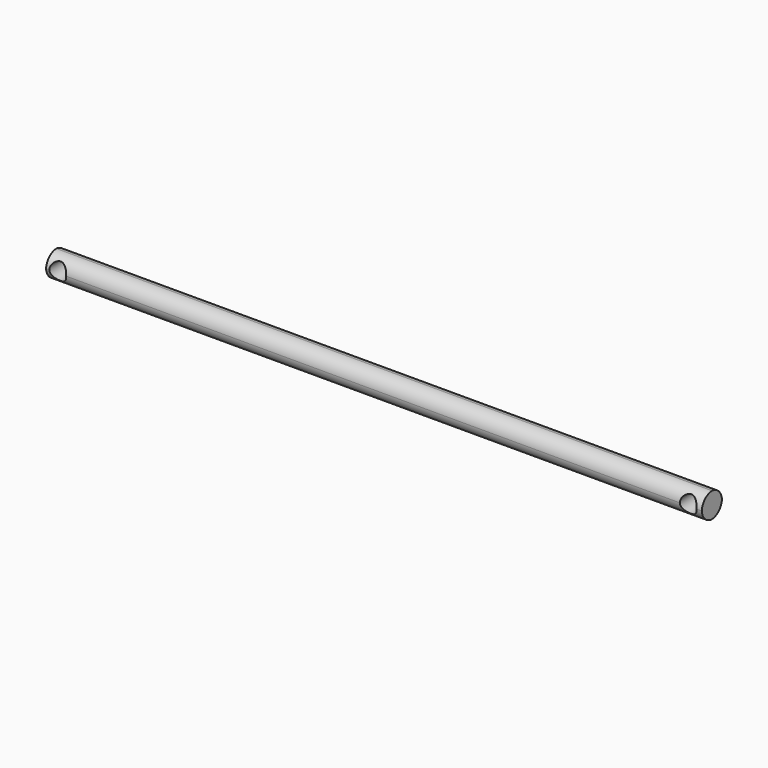
from build123d import *

# Parameters (mm, degrees)
F0_W        = 390
F0_H        = 15
F1_DEPTH    = 15
F2_R        = 5
F3_DEPTH    = 20
F4_T1_DEPTH = 430


# Not quite as in the source:
# - a fillet or chamfer that OpenCascade refuses, or shapes differently, is made with other operations: its cross-section is extruded or revolved along the edge and cut away or added


with BuildPart() as f1:
    # F0 (on Front) → F1 (new body)
    with BuildSketch(Plane.XZ):
        with Locations((-195, 7.5)):
            Rectangle(F0_W, F0_H)
    extrude(amount=F1_DEPTH)

    # F2 (on Front) → F3 (cut)
    with BuildSketch(Plane.XZ):
        with Locations((-383.0693596974, 7.6079843566)):
            Circle(F2_R)
        with Locations((-8.0693596974, 7.6553751715)):
            Circle(F2_R)
    extrude(amount=F3_DEPTH, mode=Mode.SUBTRACT)

    # F4: fillet of radius 8 on 4 edges, made by hand

    # F4_s2 → F4_t1 (cut)
    with BuildSketch(Plane.YZ.offset(-410)):
        with BuildLine():
            ThreePointArc((-8, 15), (-2.3431457505, 12.6568542495), (0, 7))
            Line((0, 7), (0, 15))
            Line((0, 15), (-8, 15))
        make_face()
        with BuildLine():
            ThreePointArc((0, 8), (-2.3431457505, 2.3431457505), (-8, 0))
            Line((-8, 0), (0, 0))
            Line((0, 0), (0, 8))
        make_face()
        with BuildLine():
            ThreePointArc((-7, 15), (-12.6568542495, 12.6568542495), (-15, 7))
            Line((-15, 7), (-15, 15))
            Line((-15, 15), (-7, 15))
        make_face()
        with BuildLine():
            ThreePointArc((-15, 8), (-12.6568542495, 2.3431457505), (-7, 0))
            Line((-7, 0), (-15, 0))
            Line((-15, 0), (-15, 8))
        make_face()
    extrude(amount=F4_T1_DEPTH, mode=Mode.SUBTRACT)


solid = f1.part
